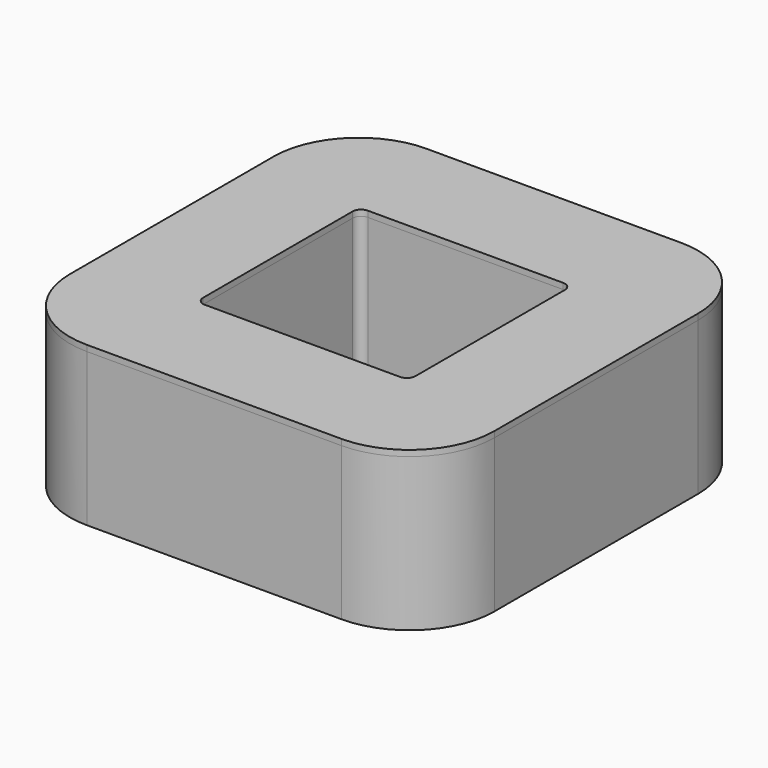
from build123d import *

# Parameters (mm, degrees)
F1_DEPTH = 18
F3_DEPTH = 18.001
F4_T     = -0.7
F6_DEPTH = 0.5
F8_DEPTH = 0.7


with BuildPart() as f1:
    # F0 (on Top) → F1 (new body)
    with BuildSketch(Plane.XY):
        with BuildLine():
            ThreePointArc((25, 15), (22.0710678119, 22.0710678119), (15, 25))
            Line((15, 25), (-15, 25))
            ThreePointArc((-15, 25), (-22.0710678119, 22.0710678119), (-25, 15))
            Line((-25, 15), (-25, -15))
            ThreePointArc((-25, -15), (-22.0710678119, -22.0710678119), (-15, -25))
            Line((-15, -25), (15, -25))
            ThreePointArc((15, -25), (22.0710678119, -22.0710678119), (25, -15))
            Line((25, -15), (25, 15))
        make_face()
    extrude(amount=F1_DEPTH)

    # F2 (on face) → F3 (cut, through all)
    with BuildSketch(Plane.XY.offset(18)):
        with BuildLine():
            ThreePointArc((12.5, 11), (12.2071067812, 11.7071067812), (11.5, 12))
            Line((11.5, 12), (-11.5, 12))
            ThreePointArc((-11.5, 12), (-12.2071067812, 11.7071067812), (-12.5, 11))
            Line((-12.5, 11), (-12.5, -11))
            ThreePointArc((-12.5, -11), (-12.2071067812, -11.7071067812), (-11.5, -12))
            Line((-11.5, -12), (11.5, -12))
            ThreePointArc((11.5, -12), (12.2071067812, -11.7071067812), (12.5, -11))
            Line((12.5, -11), (12.5, 11))
        make_face()
    extrude(amount=-F3_DEPTH, mode=Mode.SUBTRACT)

    # F4
    f4_openings = [f1.faces().sort_by_distance(p)[0] for p in [
        (24.292893, 0, 18),
    ]]
    offset(amount=F4_T, openings=f4_openings)


with BuildPart() as f6:
    # F5 (on face) → F6 (new body)
    with BuildSketch(Plane.XY.offset(18)):
        with BuildLine():
            Line((-24.05, 15), (-24.05, -15))
            ThreePointArc((-24.05, -15), (-21.3993163697, -21.3993163697), (-15, -24.05))
            Line((-15, -24.05), (15, -24.05))
            ThreePointArc((15, -24.05), (21.3993163697, -21.3993163697), (24.05, -15))
            Line((24.05, -15), (24.05, 15))
            ThreePointArc((24.05, 15), (21.3993163697, 21.3993163697), (15, 24.05))
            Line((15, 24.05), (-15, 24.05))
            ThreePointArc((-15, 24.05), (-21.3993163697, 21.3993163697), (-24.05, 15))
        make_face()
        with BuildLine():
            ThreePointArc((15, 23.5), (21.0104076401, 21.0104076401), (23.5, 15))
            Line((23.5, 15), (23.5, -15))
            ThreePointArc((23.5, -15), (21.0104076401, -21.0104076401), (15, -23.5))
            Line((15, -23.5), (-15, -23.5))
            ThreePointArc((-15, -23.5), (-21.0104076401, -21.0104076401), (-23.5, -15))
            Line((-23.5, -15), (-23.5, 15))
            ThreePointArc((-23.5, 15), (-21.0104076401, 21.0104076401), (-15, 23.5))
            Line((-15, 23.5), (15, 23.5))
        make_face(mode=Mode.SUBTRACT)
        with BuildLine():
            Line((23.5, -15), (23.5, 15))
            ThreePointArc((23.5, 15), (21.0104076401, 21.0104076401), (15, 23.5))
            Line((15, 23.5), (-15, 23.5))
            ThreePointArc((-15, 23.5), (-21.0104076401, 21.0104076401), (-23.5, 15))
            Line((-23.5, 15), (-23.5, -15))
            ThreePointArc((-23.5, -15), (-21.0104076401, -21.0104076401), (-15, -23.5))
            Line((-15, -23.5), (15, -23.5))
            ThreePointArc((15, -23.5), (21.0104076401, -21.0104076401), (23.5, -15))
        make_face()
        with BuildLine():
            ThreePointArc((11.5, 12.8), (12.7727922061, 12.2727922061), (13.3, 11))
            Line((13.3, 11), (13.3, -11))
            ThreePointArc((13.3, -11), (12.7727922061, -12.2727922061), (11.5, -12.8))
            Line((11.5, -12.8), (-11.5, -12.8))
            ThreePointArc((-11.5, -12.8), (-12.7727922061, -12.2727922061), (-13.3, -11))
            Line((-13.3, -11), (-13.3, 11))
            ThreePointArc((-13.3, 11), (-12.7727922061, 12.2727922061), (-11.5, 12.8))
            Line((-11.5, 12.8), (11.5, 12.8))
        make_face(mode=Mode.SUBTRACT)
    extrude(amount=-F6_DEPTH)

    # F7 (on face) + F6_face1 (on face) → F8 (join)
    with BuildSketch(Plane.XY.offset(18)):
        with BuildLine():
            Line((15, 25), (-15, 25))
            ThreePointArc((-15, 25), (-22.0710678119, 22.0710678119), (-25, 15))
            Line((-25, 15), (-25, -15))
            ThreePointArc((-25, -15), (-22.0710678119, -22.0710678119), (-15, -25))
            Line((-15, -25), (15, -25))
            ThreePointArc((15, -25), (22.0710678119, -22.0710678119), (25, -15))
            Line((25, -15), (25, 15))
            ThreePointArc((25, 15), (22.0710678119, 22.0710678119), (15, 25))
        make_face()
        with BuildLine():
            Line((-12.5, -11), (-12.5, 11))
            ThreePointArc((-12.5, 11), (-12.2071067812, 11.7071067812), (-11.5, 12))
            Line((-11.5, 12), (11.5, 12))
            ThreePointArc((11.5, 12), (12.2071067812, 11.7071067812), (12.5, 11))
            Line((12.5, 11), (12.5, -11))
            ThreePointArc((12.5, -11), (12.2071067812, -11.7071067812), (11.5, -12))
            Line((11.5, -12), (-11.5, -12))
            ThreePointArc((-11.5, -12), (-12.2071067812, -11.7071067812), (-12.5, -11))
        make_face(mode=Mode.SUBTRACT)
    with BuildSketch(Plane(origin=(0, 0, 17.5), x_dir=(1, 0, 0), z_dir=(0, 0, -1))):
        with BuildLine():
            Line((-15, -24.05), (15, -24.05))
            ThreePointArc((15, -24.05), (21.3993163697, -21.3993163697), (24.05, -15))
            Line((24.05, -15), (24.05, 15))
            ThreePointArc((24.05, 15), (21.3993163697, 21.3993163697), (15, 24.05))
            Line((15, 24.05), (-15, 24.05))
            ThreePointArc((-15, 24.05), (-21.3993163697, 21.3993163697), (-24.05, 15))
            Line((-24.05, 15), (-24.05, -15))
            ThreePointArc((-24.05, -15), (-21.3993163697, -21.3993163697), (-15, -24.05))
        make_face()
        with BuildLine():
            ThreePointArc((13.3, -11), (12.7727922061, -12.2727922061), (11.5, -12.8))
            Line((11.5, -12.8), (-11.5, -12.8))
            ThreePointArc((-11.5, -12.8), (-12.7727922061, -12.2727922061), (-13.3, -11))
            Line((-13.3, -11), (-13.3, 11))
            ThreePointArc((-13.3, 11), (-12.7727922061, 12.2727922061), (-11.5, 12.8))
            Line((-11.5, 12.8), (11.5, 12.8))
            ThreePointArc((11.5, 12.8), (12.7727922061, 12.2727922061), (13.3, 11))
            Line((13.3, 11), (13.3, -11))
        make_face(mode=Mode.SUBTRACT)
    extrude(amount=F8_DEPTH, dir=(0, 0, 1))


solid = Compound([f1.part, f6.part])
